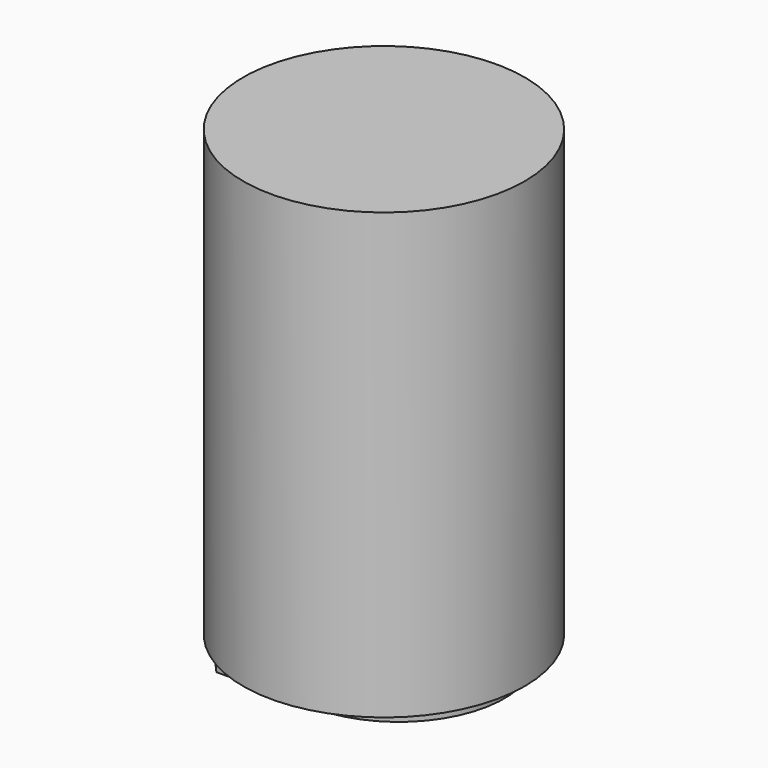
from build123d import *

# Parameters (mm, degrees)
F1_DEPTH = 2
F1_TAPER = 3
F0_R     = 9.5
F2_DEPTH = 30


with BuildPart() as f1:
    # F0 (on Top) → F1 (new body)
    with BuildSketch(Plane.XY):
        with BuildLine():
            ThreePointArc((0, -6), (7.2433005399, 1.2433005399), (0, 8.4866010798))
            Line((0, 8.4866010798), (-3.9573670752, 0))
            Line((-3.9573670752, 0), (-6.9212134549, 0))
            ThreePointArc((-6.9212134549, 0), (-7.3454775236, -0.1757359313), (-7.5212134549, -0.6))
            Line((-7.5212134549, -0.6), (-7.5212134549, -0.9))
            ThreePointArc((-7.5212134549, -0.9), (-7.3454775236, -1.3242640687), (-6.9212134549, -1.5))
            Line((-6.9212134549, -1.5), (-4.6568285624, -1.5))
            Line((-4.6568285624, -1.5), (-6.7552130241, -6))
            Line((-6.7552130241, -6), (-5.2552130241, -6))
            Line((-5.2552130241, -6), (-3.1568285624, -1.5))
            Line((-3.1568285624, -1.5), (0, -1.5))
            Line((0, -1.5), (0, -6))
        make_face()
        Polygon((0, 0), (-2.4573670752, 0), (0, 5.269840699), align=None, mode=Mode.SUBTRACT)
        with BuildLine():
            Line((1.5, -4.3006602366), (1.5, 6.7872613164))
            ThreePointArc((1.5, 6.7872613164), (5.7433005399, 1.2433005399), (1.5, -4.3006602366))
        make_face(mode=Mode.SUBTRACT)
    extrude(amount=-F1_DEPTH, taper=F1_TAPER)


with BuildPart() as f2:
    # F0 (on Top) → F2 (new body)
    with BuildSketch(Plane.XY):
        Circle(F0_R)
        with BuildLine():
            Line((-3.9573670752, 0), (0, 8.4866010798))
            ThreePointArc((0, 8.4866010798), (7.2433005399, 1.2433005399), (0, -6))
            Line((0, -6), (0, -1.5))
            Line((0, -1.5), (-3.1568285624, -1.5))
            Line((-3.1568285624, -1.5), (-5.2552130241, -6))
            Line((-5.2552130241, -6), (-6.7552130241, -6))
            Line((-6.7552130241, -6), (-4.6568285624, -1.5))
            Line((-4.6568285624, -1.5), (-6.9212134549, -1.5))
            ThreePointArc((-6.9212134549, -1.5), (-7.3454775236, -1.3242640687), (-7.5212134549, -0.9))
            Line((-7.5212134549, -0.9), (-7.5212134549, -0.6))
            ThreePointArc((-7.5212134549, -0.6), (-7.3454775236, -0.1757359313), (-6.9212134549, 0))
            Line((-6.9212134549, 0), (-3.9573670752, 0))
        make_face(mode=Mode.SUBTRACT)
        with BuildLine():
            ThreePointArc((0, -6), (7.2433005399, 1.2433005399), (0, 8.4866010798))
            Line((0, 8.4866010798), (-3.9573670752, 0))
            Line((-3.9573670752, 0), (-6.9212134549, 0))
            ThreePointArc((-6.9212134549, 0), (-7.3454775236, -0.1757359313), (-7.5212134549, -0.6))
            Line((-7.5212134549, -0.6), (-7.5212134549, -0.9))
            ThreePointArc((-7.5212134549, -0.9), (-7.3454775236, -1.3242640687), (-6.9212134549, -1.5))
            Line((-6.9212134549, -1.5), (-4.6568285624, -1.5))
            Line((-4.6568285624, -1.5), (-6.7552130241, -6))
            Line((-6.7552130241, -6), (-5.2552130241, -6))
            Line((-5.2552130241, -6), (-3.1568285624, -1.5))
            Line((-3.1568285624, -1.5), (0, -1.5))
            Line((0, -1.5), (0, -6))
        make_face()
        Polygon((0, 0), (-2.4573670752, 0), (0, 5.269840699), align=None, mode=Mode.SUBTRACT)
        with BuildLine():
            Line((1.5, -4.3006602366), (1.5, 6.7872613164))
            ThreePointArc((1.5, 6.7872613164), (5.7433005399, 1.2433005399), (1.5, -4.3006602366))
        make_face(mode=Mode.SUBTRACT)
        Polygon((0, 5.269840699), (-2.4573670752, 0), (0, 0), align=None)
        with BuildLine():
            ThreePointArc((1.5, -4.3006602366), (5.7433005399, 1.2433005399), (1.5, 6.7872613164))
            Line((1.5, 6.7872613164), (1.5, -4.3006602366))
        make_face()
    extrude(amount=F2_DEPTH)


solid = Compound([f1.part, f2.part])
